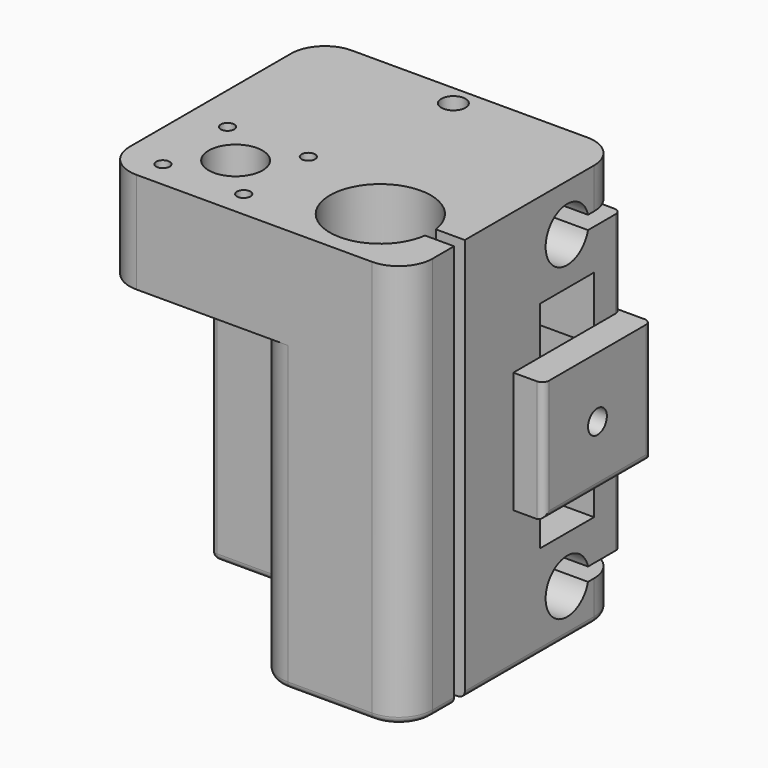
from build123d import *

# Parameters (mm, degrees)
F0_W      = 45
F0_H      = 40
F1_DEPTH  = 60
F3_W      = 10
F3_H      = 9.5
F3_H_2    = 13
F3_W_2    = 2.5
F3_W_3    = 6.1270166538
F3_H_3    = 2
F4_DEPTH  = 45
F3_W_4    = 20
F3_H_4    = 45
F5_DEPTH  = 22.5
F2_R      = 4
F2_R_2    = 1
F6_DEPTH  = 60
F7_R      = 1.75
F7_W      = 10
F7_H      = 2.5
F8_DEPTH  = 4.5
F2_R_3    = 1.8
F9_DEPTH  = 18
F10_R     = 1.8
F11_DEPTH = 18
F12_W     = 6
F12_H     = 3
F13_DEPTH = 6.5
F14_R     = 5
F15_R     = 1


# Not quite as in the source:
# - a feature names something its author has since deleted; it is built from what else it names


with BuildPart() as f1:
    # F0 (on Top) → F1 (new body)
    with BuildSketch(Plane.XY):
        with Locations((-22.5, 20)):
            Rectangle(F0_W, F0_H)
    extrude(amount=F1_DEPTH)

    # F3 (on face) → F4 (cut)
    with BuildSketch(Plane(origin=(-45, 0, 0), x_dir=(0, -1, 0), z_dir=(-1, 0, 0))):
        with BuildLine():
            Line((-33.8729833462, 54), (-33.8729833462, 52))
            ThreePointArc((-33.8729833462, 52), (-26, 53), (-33.8729833462, 54))
        make_face()
        with BuildLine():
            Line((-33.8729833462, 8), (-33.8729833462, 6))
            ThreePointArc((-33.8729833462, 6), (-26, 7), (-33.8729833462, 8))
        make_face()
        with Locations((-30, 41.25)):
            Rectangle(F3_W, F3_H)
        with Locations((-30, 30)):
            Rectangle(F3_W, F3_H_2)
        with Locations((-23.75, 30)):
            Rectangle(F3_W_2, F3_H_2)
        with Locations((-36.25, 30)):
            Rectangle(F3_W_2, F3_H_2)
        with Locations((-30, 18.75)):
            Rectangle(F3_W, F3_H)
        with Locations((-36.9364916731, 53)):
            Rectangle(F3_W_3, F3_H_3)
        with Locations((-36.9364916731, 7)):
            Rectangle(F3_W_3, F3_H_3)
    extrude(amount=-F4_DEPTH, mode=Mode.SUBTRACT)

    # F3 (on face) → F5 (cut)
    with BuildSketch(Plane(origin=(-45, 0, 0), x_dir=(0, -1, 0), z_dir=(-1, 0, 0))):
        with Locations((-10, 22.5)):
            Rectangle(F3_W_4, F3_H_4)
    extrude(amount=-F5_DEPTH, mode=Mode.SUBTRACT)

    # F2 (on face) → F6 (cut)
    with BuildSketch(Plane.XY.offset(60)):
        with Locations((-33.25, 10)):
            Circle(F2_R)
        with Locations((-27.25, 16)):
            Circle(F2_R_2)
        with Locations((-39.25, 16)):
            Circle(F2_R_2)
        with Locations((-27.25, 4)):
            Circle(F2_R_2)
        with Locations((-39.25, 4)):
            Circle(F2_R_2)
        with BuildLine():
            ThreePointArc((-4.25, 10), (-4.2667601334, 10.5011198447), (-4.3169656263, 11))
            ThreePointArc((-4.3169656263, 11), (-19.25, 10), (-4.3169656263, 9))
            ThreePointArc((-4.3169656263, 9), (-4.2667601334, 9.4988801553), (-4.25, 10))
        make_face()
        with Locations((-11.75, 10)):
            Circle(F2_R, mode=Mode.SUBTRACT)
        with Locations((-11.75, 10)):
            Circle(F2_R)
        with BuildLine():
            Line((0, 9), (0, 10))
            Line((0, 10), (-4.25, 10))
            ThreePointArc((-4.25, 10), (-4.2667601334, 9.4988801553), (-4.3169656263, 9))
            Line((-4.3169656263, 9), (0, 9))
        make_face()
        with BuildLine():
            Line((0, 10), (0, 11))
            Line((0, 11), (-4.3169656263, 11))
            ThreePointArc((-4.3169656263, 11), (-4.2667601334, 10.5011198447), (-4.25, 10))
            Line((-4.25, 10), (0, 10))
        make_face()
    extrude(amount=-F6_DEPTH, mode=Mode.SUBTRACT)

    # F7 (on face) → F8 (join)
    with BuildSketch(Plane.YZ):
        Polygon((37.5, 23.5), (37.5, 36.5), (35, 36.5), (25, 36.5), (22.5, 36.5), (22.5, 23.5), (25, 23.5), (35, 23.5), align=None)
        with Locations((30, 30)):
            Circle(F7_R, mode=Mode.SUBTRACT)
        Polygon((22.5, 36.5), (25, 36.5), (25, 39), (20, 39), (20, 21), (25, 21), (25, 23.5), (22.5, 23.5), align=None)
        with Locations((30, 37.75)):
            Rectangle(F7_W, F7_H)
        Polygon((35, 36.5), (37.5, 36.5), (37.5, 23.5), (35, 23.5), (35, 21), (40, 21), (40, 39), (35, 39), align=None)
        with Locations((30, 22.25)):
            Rectangle(F7_W, F7_H)
    extrude(amount=F8_DEPTH)

    # F2 (on face) → F9 (cut)
    with BuildSketch(Plane.XY.offset(60)):
        with Locations((-22.5, 37)):
            Circle(F2_R_3)
    extrude(amount=-F9_DEPTH, mode=Mode.SUBTRACT)

    # F10 (on face) → F11 (cut)
    with BuildSketch(Plane(origin=(0, 0, 0), x_dir=(1, 0, 0), z_dir=(0, 0, -1))):
        with Locations((-22.5, -37)):
            Circle(F10_R)
    extrude(amount=-F11_DEPTH, mode=Mode.SUBTRACT)

    # F12 (on face) → F13 (cut)
    with BuildSketch(Plane(origin=(0, 40, 0), x_dir=(-1, 0, 0), z_dir=(0, 1, 0))):
        with Locations((22.5, 45.5)):
            Rectangle(F12_W, F12_H)
        with Locations((22.5, 14.5)):
            Rectangle(F12_W, F12_H)
    extrude(amount=-F13_DEPTH, mode=Mode.SUBTRACT)

    # F14
    f14_edges = [f1.edges().sort_by_distance(p)[0] for p in [
        (-45, 0, 52.5),
        (-22.5, 0, 22.5),
        (-22.5, 20, 22.5),
        (0, 0, 30),
        (0, 40, 57),
        (0, 40, 3),
        (-45, 40, 3),
        (-45, 40, 57),
    ]]
    fillet(f14_edges, radius=F14_R)

    # F15
    f15_edges = [f1.edges().sort_by_distance(p)[0] for p in [
        (-36.25, 20, 0),
        (-22.5, 40, 0),
        (-19.25, 10, 0),
        (-45, 20, 22.5),
        (0, 40, 14.5),
        (0, 40, 45.5),
        (4.5, 40, 30),
        (4.5, 20, 30),
        (4.5, 30, 21),
        (-45, 26, 53),
        (-45, 26, 7),
        (-45, 40, 30),
    ]]
    fillet(f15_edges, radius=F15_R)


solid = f1.part
